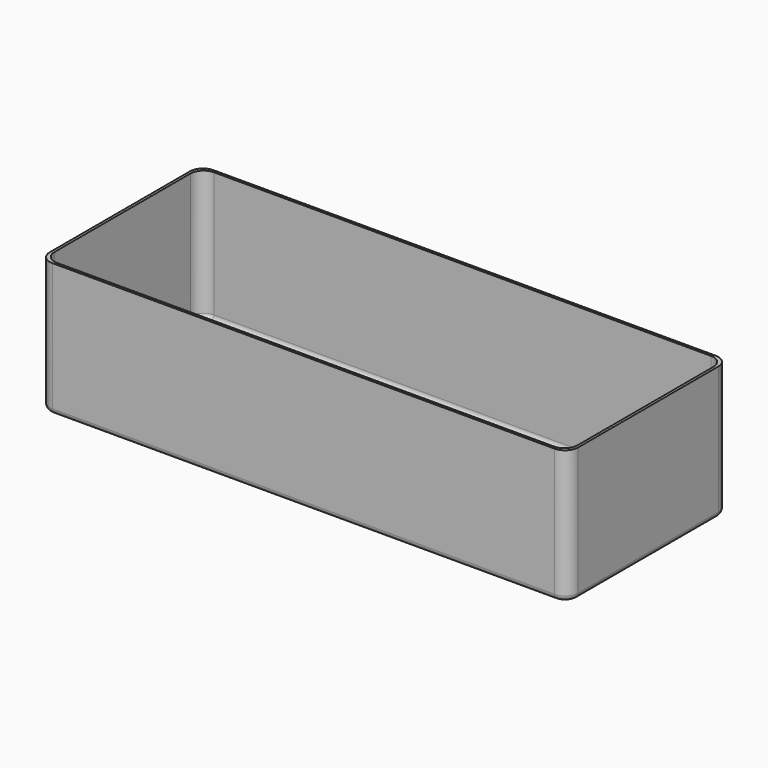
from build123d import *

# Parameters (mm, degrees)
F0_W     = 202
F0_H     = 77
F1_DEPTH = 51
F2_W     = 200
F2_H     = 75
F3_DEPTH = 50
F4_R     = 5
F5_R     = 2


# Not quite as in the source:
# - a feature of the source that left no trace in its solid (it failed there, or was rolled back) is left out


with BuildPart() as f1:
    # F0 (on Top) → F1 (new body)
    with BuildSketch(Plane.XY):
        with Locations((-2.8100872189, -1.361513185)):
            Rectangle(F0_W, F0_H)
    extrude(amount=F1_DEPTH)

    # F2 (on face) → F3 (cut)
    with BuildSketch(Plane.XY.offset(51)):
        with Locations((-2.8100872189, -1.361513185)):
            Rectangle(F2_W, F2_H)
    extrude(amount=-F3_DEPTH, mode=Mode.SUBTRACT)

    # F4
    f4_edges = [f1.edges().sort_by_distance(p)[0] for p in [
        (97.189913, 36.138487, 26),
        (-102.810087, 36.138487, 26),
        (97.189913, -38.861513, 26),
        (-102.810087, -38.861513, 26),
        (98.189913, 37.138487, 25.5),
        (-103.810087, 37.138487, 25.5),
        (98.189913, -39.861513, 25.5),
        (-103.810087, -39.861513, 25.5),
    ]]
    fillet(f4_edges, radius=F4_R)

    # F5
    f5_edges = [f1.edges().sort_by_distance(p)[0] for p in [
        (97.189913, -1.361513, 1),
        (-2.810087, 36.138487, 1),
        (-2.810087, -38.861513, 1),
        (-2.810087, 37.138487, 0),
        (96.725447, 35.674021, 0),
        (-102.345621, 35.674021, 0),
        (98.189913, -1.361513, 0),
        (-103.810087, -1.361513, 0),
        (96.725447, -38.397047, 0),
        (-102.345621, -38.397047, 0),
        (-2.810087, -39.861513, 0),
        (95.725447, -37.397047, 1),
        (95.725447, 34.674021, 1),
        (-101.345621, -37.397047, 1),
        (-101.345621, 34.674021, 1),
        (-102.810087, -1.361513, 1),
    ]]
    fillet(f5_edges, radius=F5_R)


solid = f1.part
